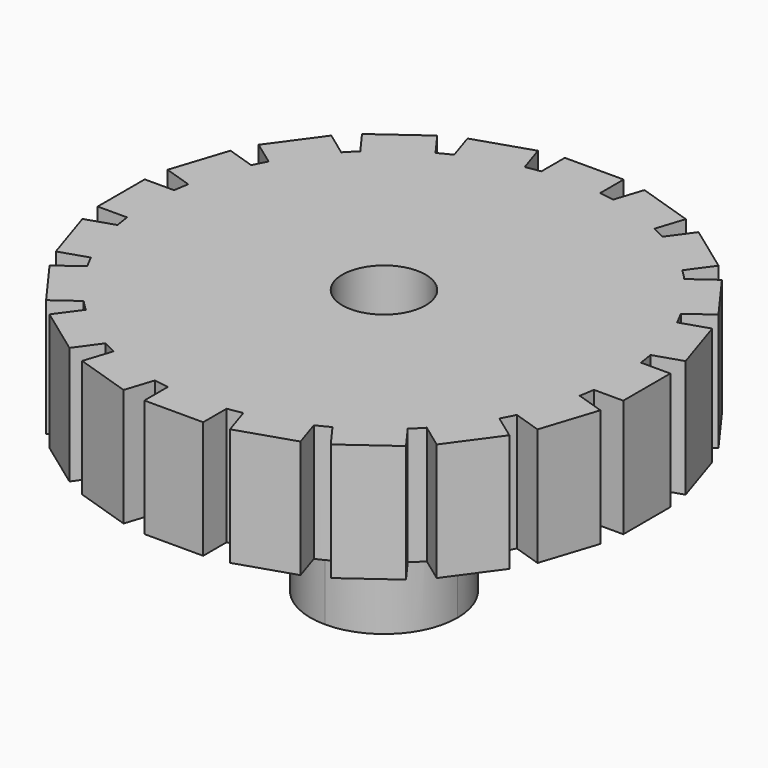
from build123d import *

# Parameters (mm, degrees)
F0_R        = 12.7
F0_R_2      = 2.2479
F1_DEPTH    = 6.35
F2_W        = 7.9375
F2_H        = 7.9375
F2_R        = 2.2479
F3_DEPTH    = 7.9375
F5_REACH    = 20.5318866107
F6_T1_DEPTH = 17.859375
F7_W        = 1.5875
F7_H        = 3.175
F8_DEPTH    = 6.35
F9_COUNT    = 20
F9_ANGLE    = 342


# Not quite as in the source:
# - a fillet or chamfer that OpenCascade refuses, or shapes differently, is made with other operations: its cross-section is extruded or revolved along the edge and cut away or added


with BuildPart() as f1:
    # F0 (on Top) → F1 (new body)
    with BuildSketch(Plane.XY):
        Circle(F0_R)
        Circle(F0_R_2, mode=Mode.SUBTRACT)
    extrude(amount=F1_DEPTH)

    # F2 (on face) → F3 (join)
    with BuildSketch(Plane(origin=(0, 0, 0), x_dir=(1, 0, 0), z_dir=(0, 0, -1))):
        Rectangle(F2_W, F2_H)
        Circle(F2_R, mode=Mode.SUBTRACT)
    extrude(amount=F3_DEPTH)

    f5_end = f1.faces().sort_by_distance((-2.2479, 0, -0.79375))[0]
    # F4 (on face) → F5 (cut, up to a face of the model that its end follows)
    with BuildSketch(Plane.YZ.offset(3.96875)):
        with BuildLine():
            ThreePointArc((-1.7272, -3.96875), (0, -5.69595), (1.7272, -3.96875))
            Line((1.7272, -3.96875), (-1.7272, -3.96875))
        make_face()
        with BuildLine():
            Line((-1.7272, -3.96875), (1.7272, -3.96875))
            ThreePointArc((1.7272, -3.96875), (0, -2.24155), (-1.7272, -3.96875))
        make_face()
    f5_long = extrude(amount=-F5_REACH, mode=Mode.PRIVATE)
    add(split(f5_long, bisect_by=f5_end, keep=Keep.ALL, mode=Mode.PRIVATE).solids().sort_by_distance((3.96875, 0, -3.96875))[0], mode=Mode.SUBTRACT)

    # F6: fillet of radius 3.96875 on 4 edges, made by hand

    # F6_s2 → F6_t1 (cut)
    with BuildSketch(Plane.XY.offset(-17.859375)):
        with BuildLine():
            ThreePointArc((0, 3.96875), (2.8063300378, 2.8063300378), (3.96875, 0))
            Line((3.96875, 0), (3.96875, 3.96875))
            Line((3.96875, 3.96875), (0, 3.96875))
        make_face()
        with BuildLine():
            ThreePointArc((0, 3.96875), (-2.8063300378, 2.8063300378), (-3.96875, 0))
            Line((-3.96875, 0), (-3.96875, 3.96875))
            Line((-3.96875, 3.96875), (0, 3.96875))
        make_face()
        with BuildLine():
            ThreePointArc((-3.96875, 0), (-2.8063300378, -2.8063300378), (0, -3.96875))
            Line((0, -3.96875), (-3.96875, -3.96875))
            Line((-3.96875, -3.96875), (-3.96875, 0))
        make_face()
        with BuildLine():
            ThreePointArc((0, -3.96875), (2.8063300378, -2.8063300378), (3.96875, 0))
            Line((3.96875, 0), (3.96875, -3.96875))
            Line((3.96875, -3.96875), (0, -3.96875))
        make_face()
    extrude(amount=F6_T1_DEPTH, mode=Mode.SUBTRACT)

    # F7 (on face) → F8 (join, through all)
    with BuildSketch(Plane.XY.offset(6.35)):
        with Locations((13.3941406189, 0)):
            Rectangle(F7_W, F7_H)
    f8 = extrude(amount=-F8_DEPTH)

    # F9: F8 ×20 about axis
    f9_axis = Axis((0, 0, 0), (0, 0, -1))
    for i in range(1, F9_COUNT):
        add(f8.rotate(f9_axis, i * F9_ANGLE / (F9_COUNT - 1)))


solid = f1.part
